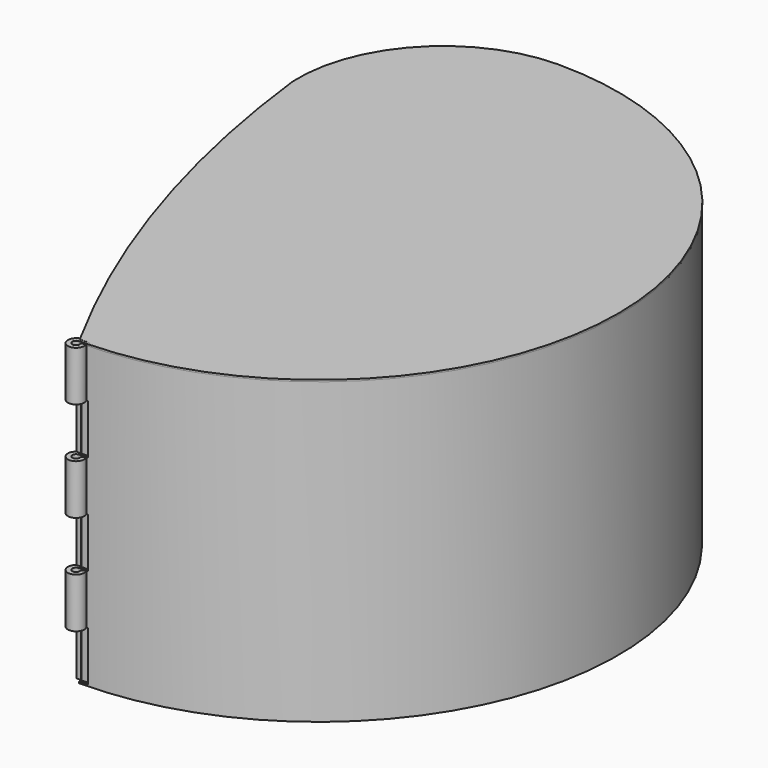
from build123d import *

# Parameters (mm, degrees)
F1_DEPTH      = 0.889
F3_DEPTH      = 152.4
F5_DEPTH      = 152.4
F7_DEPTH      = 2.794
F7_DEPTH_BACK = 25.4


with BuildPart() as f1:
    # F0 (on Top) → F1 (new body)
    with BuildSketch(Plane.XY):
        with BuildLine():
            Line((104.8647104191, 103.4104977604), (107.4410535939, 105.9511134646))
            ThreePointArc((107.4410535939, 105.9511134646), (57.5440925804, 139.9647071727), (-1.646224697, 151.9287205432))
            ThreePointArc((-1.646224697, 151.9287205432), (-54.8274165052, 128.8286295835), (-74.9656821683, 74.4567285632))
            ThreePointArc((-74.9656821683, 74.4567285632), (-50.0786323185, -40.6329360959), (-3.82113499, -148.9160839189))
            ThreePointArc((-3.82113499, -148.9160839189), (134.5057048325, -58.9275907244), (104.8647104191, 103.4104977604))
        make_face()
        with BuildLine():
            ThreePointArc((-3.82113499, -148.9160839189), (-2.7372897039, -150.8956667029), (-1.646224697, -152.8712794568))
            ThreePointArc((-1.646224697, -152.8712794568), (138.7897619326, -59.6615967341), (107.4410535939, 105.9511134646))
            Line((107.4410535939, 105.9511134646), (104.8647104191, 103.4104977604))
            ThreePointArc((104.8647104191, 103.4104977604), (134.5057048325, -58.9275907244), (-3.82113499, -148.9160839189))
        make_face()
    extrude(amount=F1_DEPTH)

    # F4 (on face) → F5 (join)
    with BuildSketch(Plane.XY.offset(0.889)):
        with BuildLine():
            ThreePointArc((0.0687806999, -154.0492904087), (-2.6435357958, -156.5016984542), (-1.681308085, -152.9739394166))
            Line((-1.681308085, -152.9739394166), (-1.681308085, -152.8080176611))
            ThreePointArc((-1.681308085, -152.8080176611), (-2.2202251071, -151.834050614), (-2.7573875275, -150.8591147702))
            ThreePointArc((-2.7573875275, -150.8591147702), (-3.3669851054, -158.6773081165), (2.108116449, -153.0631279113))
            Line((2.108116449, -153.0631279113), (0.0687806999, -154.0492904087))
        make_face()
        with BuildLine():
            ThreePointArc((-2.7573875275, -150.8591147702), (-2.2202251071, -151.834050614), (-1.681308085, -152.8080176611))
            Line((-1.681308085, -152.8080176611), (-1.681308085, -150.7085030485))
            ThreePointArc((-1.681308085, -150.7085030485), (-2.2242740643, -150.7486121468), (-2.7573875275, -150.8591147702))
        make_face()
    extrude(amount=-F5_DEPTH)


with BuildPart() as f3:
    # F2 (on face) → F3 (new body)
    with BuildSketch(Plane(origin=(0, 0, 0), x_dir=(1, 0, 0), z_dir=(0, 0, -1))):
        with BuildLine():
            Line((89.605505981, -118.7772235698), (90.8628587214, -120.4439165471))
            ThreePointArc((90.8628587214, -120.4439165471), (142.4534143114, 49.3313434088), (-1.646224697, 152.8712794568))
            Line((-1.646224697, 152.8712794568), (-1.646224697, 150.7014483213))
            ThreePointArc((-1.646224697, 150.7014483213), (140.2771274439, 48.5706756767), (89.605505981, -118.7772235698))
        make_face()
    extrude(amount=F3_DEPTH)


with BuildPart() as f7_tool:
    # F6 (on Right) → F7 (new body, two sides)
    with BuildSketch(Plane.YZ) as f7_sk:
        Polygon((-160.2078721456, 0.8427356878), (-151.5557976027, 0.8427356878), (-151.5557976027, 9.4913730934), (-177.3275714077, 9.4913730934), (-177.3275714077, -151.5572643122), (-151.5557976027, -151.5572643122), (-151.5557976027, -126.1572643122), (-160.2078721456, -126.1572643122), (-160.2078721456, -100.7572643122), (-151.5557976027, -100.7572643122), (-151.5557976027, -75.3572643122), (-160.2078721456, -75.3572643122), (-160.2078721456, -49.9572643122), (-151.5557976027, -49.9572643122), (-151.5557976027, -24.5572643122), (-160.2078721456, -24.5572643122), align=None)
    extrude(amount=F7_DEPTH)
    extrude(f7_sk.sketch, amount=-F7_DEPTH_BACK)


with BuildPart() as f1_1:
    add(f1.part)

    # F7: cut by f7_tool
    add(f7_tool.part, mode=Mode.SUBTRACT)


with BuildPart() as f3_1:
    add(f3.part)

    # F7: cut by f7_tool
    add(f7_tool.part, mode=Mode.SUBTRACT)


solid = Compound([f1_1.part, f3_1.part])
